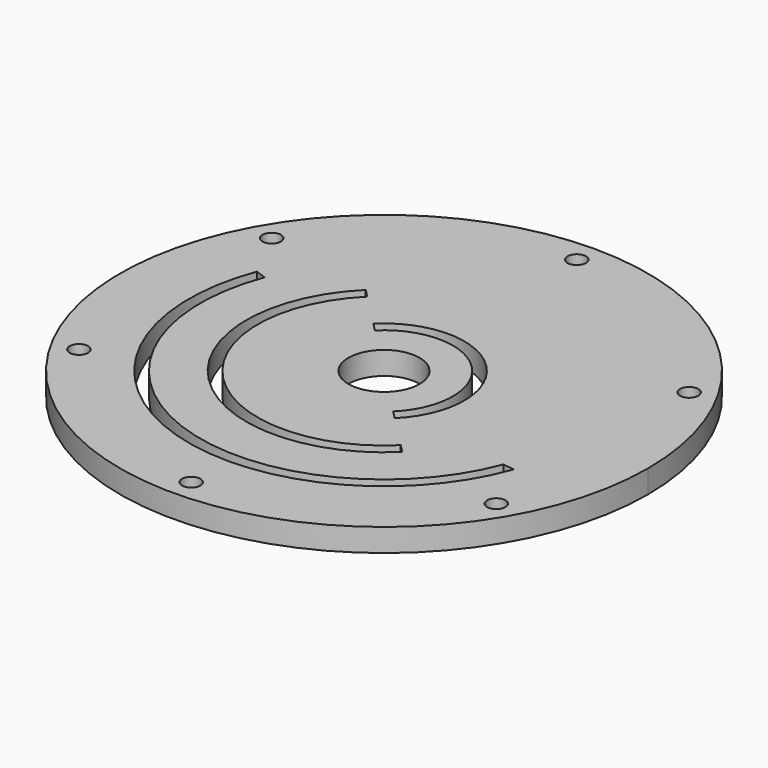
from build123d import *

# Parameters (mm, degrees)
F0_R            = 15.5
F1_DEPTH        = 10
F2_R            = 4
F3_DEPTH        = 25
F3_COPIES_COUNT = 6


# Not quite as in the source:
# - a pattern or mirror of a feature is missing from the dataset's text; its kind, count and spacing are read off the source's solid


with BuildPart() as f1:
    # F0 (on Top) → F1 (new body)
    with BuildSketch(Plane.XY):
        with BuildLine():
            ThreePointArc((115, 0), (81.3172798365, 81.3172798365), (0, 115))
            ThreePointArc((0, 115), (-81.3172798365, -81.3172798365), (115, 0))
        make_face()
        with BuildLine():
            ThreePointArc((79.8738727668, -29.0717121827), (-29.6258097027, -79.6700156863), (-79.4623147975, 30.1784778779))
            Line((-79.4623147975, 30.1784778779), (-74.7757231643, 28.4357385213))
            ThreePointArc((-74.7757231643, 28.4357385213), (-28.4357385213, -74.7757231643), (74.7757231643, -28.4357385213))
            Line((74.7757231643, -28.4357385213), (79.8738727668, -29.0717121827))
        make_face(mode=Mode.SUBTRACT)
        with BuildLine():
            Line((-42.1306922898, 42.7200745222), (-38.6198012657, 39.160068312))
            ThreePointArc((-38.6198012657, 39.160068312), (-39.160068312, -38.6198012657), (38.6198012657, -39.160068312))
            Line((38.6198012657, -39.160068312), (42.1306922898, -42.7200745222))
            ThreePointArc((42.1306922898, -42.7200745222), (-42.7200745222, -42.1306922898), (-42.1306922898, 42.7200745222))
        make_face(mode=Mode.SUBTRACT)
        Circle(F0_R, mode=Mode.SUBTRACT)
        with BuildLine():
            ThreePointArc((-24.5762371691, 24.9200434713), (24.9200434713, 24.5762371691), (24.5762371691, -24.9200434713))
            Line((24.5762371691, -24.9200434713), (21.0653461449, -21.3600372611))
            ThreePointArc((21.0653461449, -21.3600372611), (21.3600372611, 21.0653461449), (-21.0653461449, 21.3600372611))
            Line((-21.0653461449, 21.3600372611), (-24.5762371691, 24.9200434713))
        make_face(mode=Mode.SUBTRACT)
    extrude(amount=F1_DEPTH)

    # F2 (on face) → F3 (cut)
    with BuildSketch(Plane.XY.offset(10)):
        with Locations((0, 105)):
            Circle(F2_R)
    f3 = extrude(amount=-F3_DEPTH, mode=Mode.SUBTRACT)

    # F3_copies: F3 ×6 about axis
    f3_copies_axis = Axis((0, 0, 0), (0, 0, 1))
    for i in range(1, F3_COPIES_COUNT):
        add(f3.rotate(f3_copies_axis, i * 360 / F3_COPIES_COUNT), mode=Mode.SUBTRACT)


solid = f1.part
